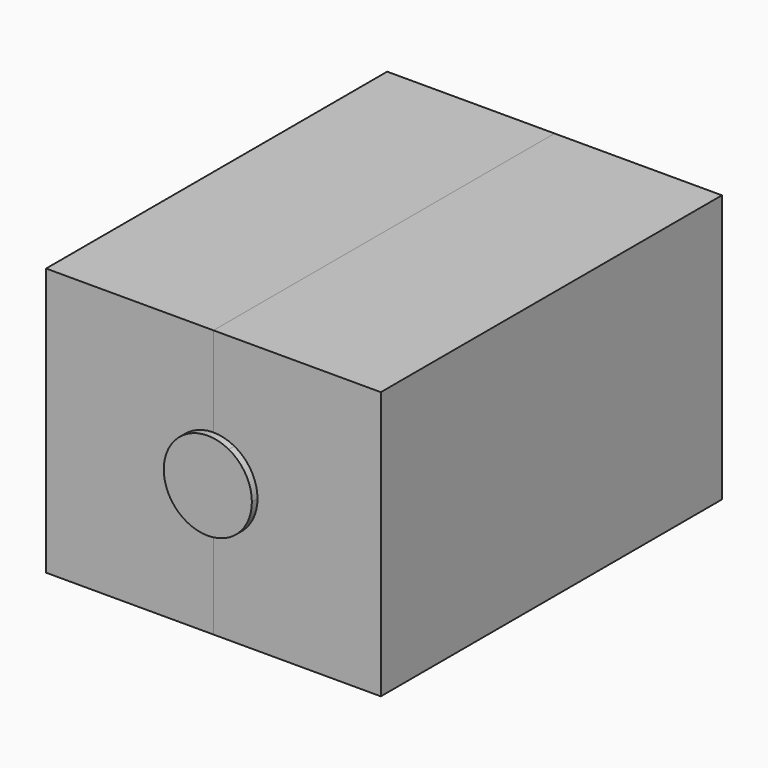
from build123d import *

# Parameters (mm, degrees)
F1_DEPTH  = 10.795
F0_W      = 11.557
F0_H      = 2.286
F2_DEPTH  = 6.604
F3_DEPTH  = 7.62
F0_W_2    = 10.922
F0_H_2    = 5.588
F0_W_3    = 0.508
F4_DEPTH  = 6.35
F0_W_4    = 1.016
F5_DEPTH  = 4.699
F7_DEPTH  = 2.54
F8_DEPTH  = 1.016
F9_DEPTH  = 12.065
F10_DEPTH = 12.065


with BuildPart() as f1:
    # F0 (on Right) → F1 (new body, symmetric)
    with BuildSketch(Plane.YZ):
        Polygon((0, -2.032), (0, 0), (-1.905, 0), (-12.827, 0), (-12.827, -2.032), (-11.557, -2.032), align=None)
        Polygon((12.827, 0), (0, 0), (0, -2.032), (11.557, -2.032), (12.827, -2.032), align=None)
    extrude(amount=F1_DEPTH, both=True)

    # F0 (on Right) → F2 (join, symmetric)
    with BuildSketch(Plane.YZ):
        with Locations((-5.7785, -3.175)):
            Rectangle(F0_W, F0_H)
        with Locations((5.7785, -3.175)):
            Rectangle(F0_W, F0_H)
    extrude(amount=F2_DEPTH, both=True)

    # F0 (on Right) → F3 (join, symmetric)
    with BuildSketch(Plane.YZ):
        Polygon((-1.905, 0), (0, 0), (12.827, 0), (14.351, 0), (14.351, 9.906), (-1.905, 9.906), (-1.905, 5.588), align=None)
    extrude(amount=F3_DEPTH, both=True)

    # F0 (on Right) → F4 (join, symmetric)
    with BuildSketch(Plane.YZ):
        with Locations((-7.366, 2.794)):
            Rectangle(F0_W_2, F0_H_2)
        with Locations((-13.081, 2.794)):
            Rectangle(F0_W_3, F0_H_2)
    extrude(amount=F4_DEPTH, both=True)

    # F0 (on Right) → F5 (join, symmetric)
    with BuildSketch(Plane.YZ):
        with Locations((-13.843, 2.794)):
            Rectangle(F0_W_4, F0_H_2)
    extrude(amount=F5_DEPTH, both=True)

    # F6 (on face) → F8 (join)
    with BuildSketch(Plane.XZ.offset(14.351)):
        with BuildLine():
            Line((1.5080414451, 5.588), (0, 5.588))
            Line((0, 5.588), (0, 0))
            Line((0, 0), (1.5080414451, 0))
            ThreePointArc((1.5080414451, 0), (2.726596467, 1.1672557958), (3.175, 2.794))
            ThreePointArc((3.175, 2.794), (2.726596467, 4.4207442042), (1.5080414451, 5.588))
        make_face()
        with BuildLine():
            Line((-1.5080414451, 5.588), (0, 5.588))
            Line((0, 5.588), (1.5080414451, 5.588))
            ThreePointArc((1.5080414451, 5.588), (0, 5.969), (-1.5080414451, 5.588))
        make_face()
        with BuildLine():
            Line((1.5080414451, 0), (0, 0))
            Line((0, 0), (-1.5080414451, 0))
            ThreePointArc((-1.5080414451, 0), (0, -0.381), (1.5080414451, 0))
        make_face()
    extrude(amount=-F8_DEPTH)


with BuildPart() as f7:
    # F6 (on face) → F7 (new body)
    with BuildSketch(Plane.XZ.offset(14.351)):
        with BuildLine():
            Line((1.5080414451, 5.588), (0, 5.588))
            Line((0, 5.588), (0, 0))
            Line((0, 0), (1.5080414451, 0))
            ThreePointArc((1.5080414451, 0), (2.726596467, 1.1672557958), (3.175, 2.794))
            ThreePointArc((3.175, 2.794), (2.726596467, 4.4207442042), (1.5080414451, 5.588))
        make_face()
        with BuildLine():
            Line((-1.5080414451, 5.588), (0, 5.588))
            Line((0, 5.588), (1.5080414451, 5.588))
            ThreePointArc((1.5080414451, 5.588), (0, 5.969), (-1.5080414451, 5.588))
        make_face()
        with BuildLine():
            Line((0, 0), (0, 5.588))
            Line((0, 5.588), (-1.5080414451, 5.588))
            ThreePointArc((-1.5080414451, 5.588), (-3.175, 2.794), (-1.5080414451, 0))
            Line((-1.5080414451, 0), (0, 0))
        make_face()
        with BuildLine():
            Line((1.5080414451, 0), (0, 0))
            Line((0, 0), (-1.5080414451, 0))
            ThreePointArc((-1.5080414451, 0), (0, -0.381), (1.5080414451, 0))
        make_face()
    extrude(amount=F7_DEPTH)


with BuildPart() as f9:
    # F0 (on Right) → F9 (new body)
    with BuildSketch(Plane.YZ):
        Polygon((-12.827, 5.588), (-1.905, 5.588), (-1.905, 9.906), (14.351, 9.906), (14.351, 12.446), (-16.383, 12.446), (-16.383, 0), (-14.351, 0), (-14.351, 5.588), (-13.335, 5.588), align=None)
        Polygon((-12.827, -2.032), (-12.827, 0), (-13.335, 0), (-14.351, 0), (-16.383, 0), (-16.383, -6.858), (-11.557, -6.858), (-11.557, -4.318), (-11.557, -2.032), align=None)
        Polygon((14.351, 0), (12.827, 0), (12.827, -2.032), (11.557, -2.032), (11.557, -4.318), (0, -4.318), (-11.557, -4.318), (-11.557, -6.858), (14.351, -6.858), align=None)
        with Locations((-13.843, 2.794)):
            Rectangle(F0_W_4, F0_H_2)
        with Locations((-7.366, 2.794)):
            Rectangle(F0_W_2, F0_H_2)
        with Locations((-13.081, 2.794)):
            Rectangle(F0_W_3, F0_H_2)
        Polygon((0, -2.032), (0, 0), (-1.905, 0), (-12.827, 0), (-12.827, -2.032), (-11.557, -2.032), align=None)
        with Locations((-5.7785, -3.175)):
            Rectangle(F0_W, F0_H)
        with Locations((5.7785, -3.175)):
            Rectangle(F0_W, F0_H)
        Polygon((12.827, 0), (0, 0), (0, -2.032), (11.557, -2.032), (12.827, -2.032), align=None)
        Polygon((-1.905, 0), (0, 0), (12.827, 0), (14.351, 0), (14.351, 9.906), (-1.905, 9.906), (-1.905, 5.588), align=None)
    extrude(amount=F9_DEPTH)

    # F11: cut F1, F7
    add(f1.part, mode=Mode.SUBTRACT)
    add(f7.part, mode=Mode.SUBTRACT)


with BuildPart() as f10:
    # F0 (on Right) → F10 (new body)
    with BuildSketch(Plane.YZ):
        Polygon((-12.827, 5.588), (-1.905, 5.588), (-1.905, 9.906), (14.351, 9.906), (14.351, 12.446), (-16.383, 12.446), (-16.383, 0), (-14.351, 0), (-14.351, 5.588), (-13.335, 5.588), align=None)
        Polygon((-1.905, 0), (0, 0), (12.827, 0), (14.351, 0), (14.351, 9.906), (-1.905, 9.906), (-1.905, 5.588), align=None)
        with Locations((-7.366, 2.794)):
            Rectangle(F0_W_2, F0_H_2)
        with Locations((-13.081, 2.794)):
            Rectangle(F0_W_3, F0_H_2)
        with Locations((-13.843, 2.794)):
            Rectangle(F0_W_4, F0_H_2)
        Polygon((-12.827, -2.032), (-12.827, 0), (-13.335, 0), (-14.351, 0), (-16.383, 0), (-16.383, -6.858), (-11.557, -6.858), (-11.557, -4.318), (-11.557, -2.032), align=None)
        Polygon((0, -2.032), (0, 0), (-1.905, 0), (-12.827, 0), (-12.827, -2.032), (-11.557, -2.032), align=None)
        with Locations((-5.7785, -3.175)):
            Rectangle(F0_W, F0_H)
        Polygon((14.351, 0), (12.827, 0), (12.827, -2.032), (11.557, -2.032), (11.557, -4.318), (0, -4.318), (-11.557, -4.318), (-11.557, -6.858), (14.351, -6.858), align=None)
        with Locations((5.7785, -3.175)):
            Rectangle(F0_W, F0_H)
        Polygon((12.827, 0), (0, 0), (0, -2.032), (11.557, -2.032), (12.827, -2.032), align=None)
    extrude(amount=-F10_DEPTH)

    # F11: cut F1, F7
    add(f1.part, mode=Mode.SUBTRACT)
    add(f7.part, mode=Mode.SUBTRACT)


solid = Compound([f1.part, f7.part, f9.part, f10.part])
